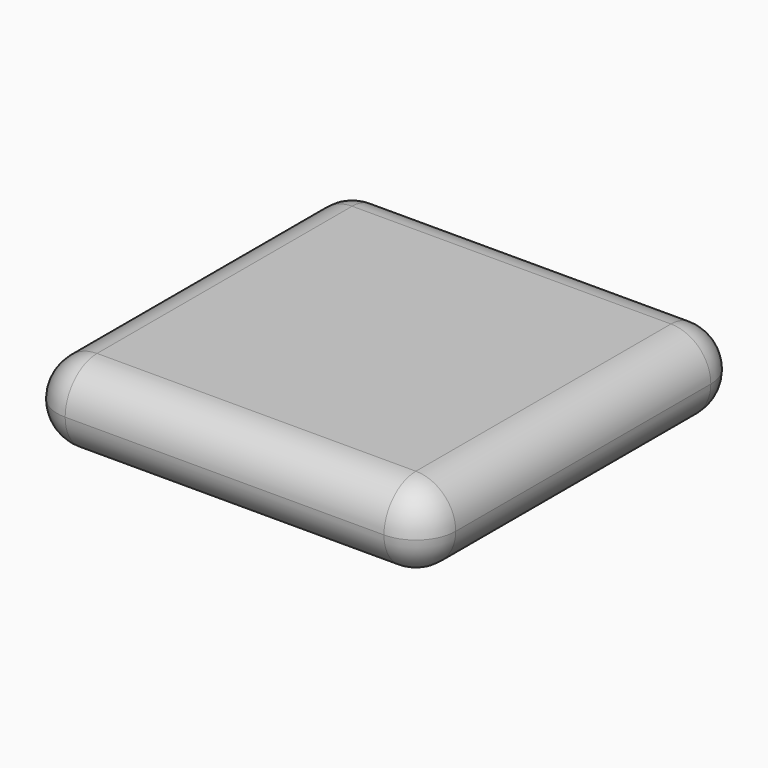
from build123d import *

# Parameters (mm, degrees)
F0_W     = 100
F0_H     = 100
F1_DEPTH = 20
F2_R     = 9.99999


# Not quite as in the source:
# - a fillet or chamfer is up to 0.001 mm smaller than in the source, because OpenCascade refuses the exact size


with BuildPart() as f1:
    # F0 (on Top) → F1 (new body)
    with BuildSketch(Plane.XY):
        with Locations((50, 50)):
            Rectangle(F0_W, F0_H)
    extrude(amount=F1_DEPTH)

    # F2 (radius 10 in the source; OpenCascade refuses exactly that, so slightly less here)
    f2_edges = [f1.edges().sort_by_distance(p)[0] for p in [
        (100, 0, 10),
        (100, 100, 10),
        (100, 50, 0),
        (100, 50, 20),
        (0, 100, 10),
        (50, 100, 0),
        (50, 100, 20),
        (0, 0, 10),
        (0, 50, 0),
        (0, 50, 20),
        (50, 0, 0),
        (50, 0, 20),
    ]]
    fillet(f2_edges, radius=F2_R)


solid = f1.part
